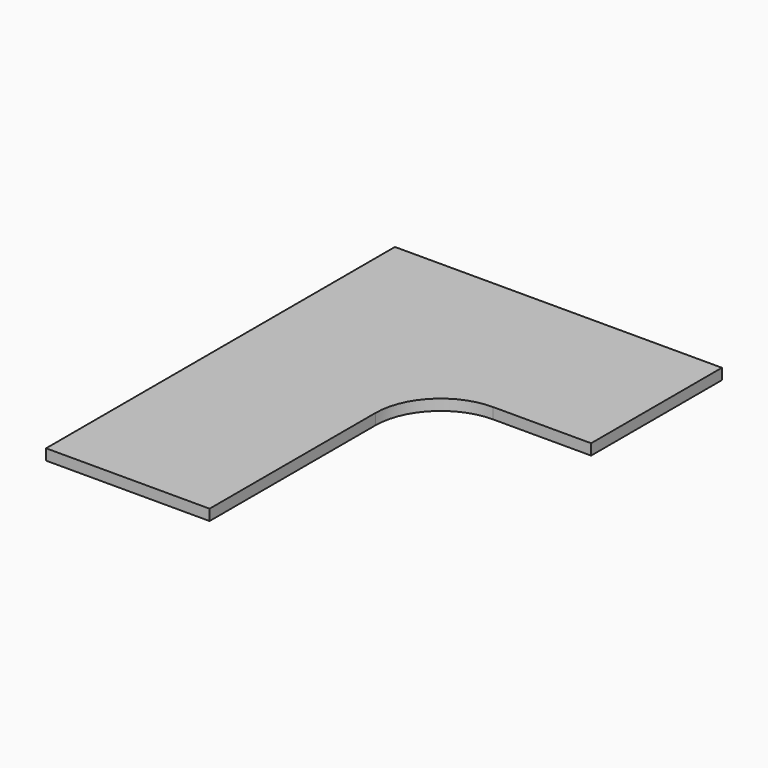
from build123d import *

# Parameters (mm, degrees)
F9_DEPTH = 50


# Not quite as in the source:
# - the program builds the solid bodies; features that only make, move or delete a surface that nothing else refers to are left out


with BuildPart() as f9:
    # F3 (on offset) → F9 (new body)
    with BuildSketch(Plane.XY.offset(750)):
        with BuildLine():
            ThreePointArc((0, -300), (87.867965644, -87.867965644), (300, 0))
            Line((300, 0), (750, 0))
            Line((750, 0), (750, 750))
            Line((750, 750), (-750, 750))
            Line((-750, 750), (-750, -1250))
            Line((-750, -1250), (0, -1250))
            Line((0, -1250), (0, -300))
        make_face()
    extrude(amount=-F9_DEPTH)


solid = f9.part
